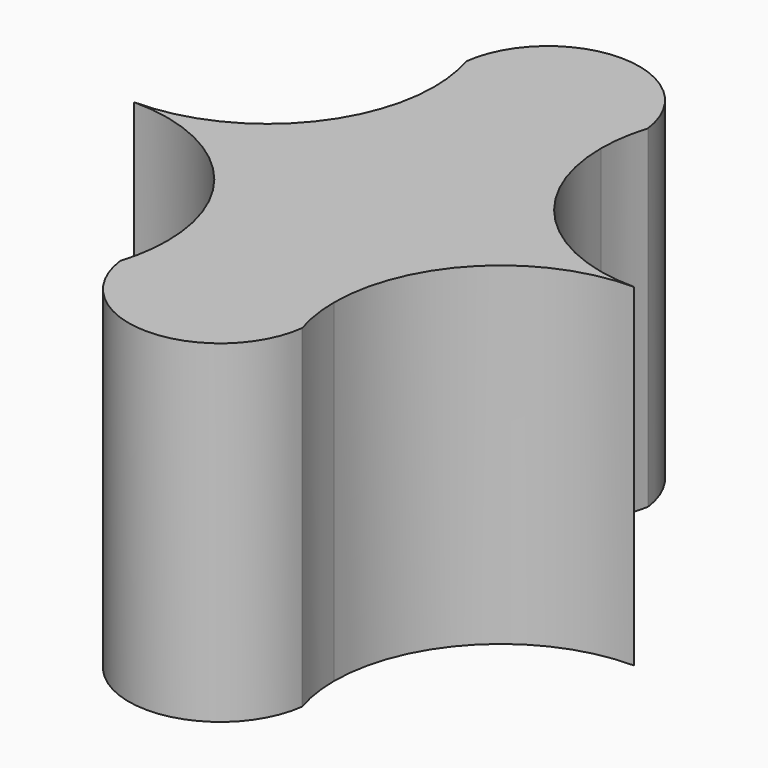
from build123d import *

# Parameters (mm, degrees)
F1_DEPTH = 25.4


# Not quite as in the source:
# - a feature names something its author has since deleted; it is built from what else it names


with BuildPart() as f1:
    # F0 (on Top) → F1 (new body)
    with BuildSketch(Plane.XY):
        with BuildLine():
            ThreePointArc((-6.920715507, 16.4643668374), (-6.4934894763, 14.6036920626), (-6.35, 12.7))
            Line((-6.35, 12.7), (6.35, 12.7))
            ThreePointArc((6.35, 12.7), (6.4934894763, 14.6036920626), (6.920715507, 16.4643668374))
            ThreePointArc((6.920715507, 16.4643668374), (0, 22.5641302142), (-6.920715507, 16.4643668374))
        make_face()
        with BuildLine():
            Line((6.35, 12.7), (-6.35, 12.7))
            ThreePointArc((-6.35, 12.7), (-10.0697438789, 3.7197438789), (-19.05, 0))
            ThreePointArc((-19.05, 0), (-10.0697438789, -3.7197438789), (-6.35, -12.7))
            Line((-6.35, -12.7), (6.35, -12.7))
            ThreePointArc((6.35, -12.7), (10.0697438789, -3.7197438789), (19.05, 0))
            ThreePointArc((19.05, 0), (10.0697438789, 3.7197438789), (6.35, 12.7))
        make_face()
        with BuildLine():
            Line((6.35, -12.7), (-6.35, -12.7))
            ThreePointArc((-6.35, -12.7), (-6.4956231596, -14.6177127391), (-6.9291530945, -16.4914469919))
            ThreePointArc((-6.9291530945, -16.4914469919), (0, -22.5949355663), (6.9291530945, -16.4914469919))
            ThreePointArc((6.9291530945, -16.4914469919), (6.4956231596, -14.6177127391), (6.35, -12.7))
        make_face()
    extrude(amount=F1_DEPTH)


solid = f1.part
